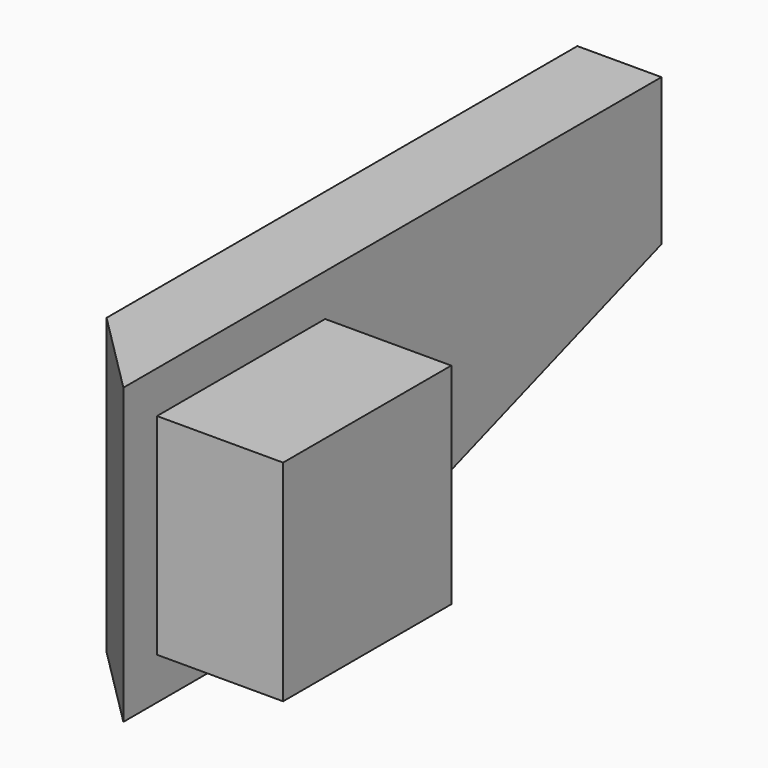
from build123d import *

# Parameters (mm, degrees)
F0_W     = 5
F0_H     = 5
F1_DEPTH = 3
F2_W     = 5
F2_H     = 5
F3_DEPTH = 2
F4_SIZE  = 1.99999


# Not quite as in the source:
# - a fillet or chamfer is up to 0.001 mm smaller than in the source, because OpenCascade refuses the exact size


with BuildPart() as f1:
    # F0 (on Right) → F1 (new body)
    with BuildSketch(Plane.YZ):
        with Locations((40.6040474772, 32.0952650385)):
            Rectangle(F0_W, F0_H)
    extrude(amount=F1_DEPTH)

    # F2 (on face) → F3 (join)
    with BuildSketch(Plane(origin=(0, 0, 0), x_dir=(0, -1, 0), z_dir=(-1, 0, 0))):
        with Locations((-40.6040474772, 32.0952650385)):
            Rectangle(F2_W, F2_H)
        Polygon((-37.1040474772, 28.5952650385), (-37.1040474772, 35.5952650385), (-43.1040474772, 35.5952650385), (-43.1040474772, 34.5952650385), (-38.1040474772, 34.5952650385), (-38.1040474772, 29.5952650385), (-43.1040474772, 29.5952650385), (-43.1040474772, 28.5952650385), align=None)
        Polygon((-43.1040474772, 34.5952650385), (-43.1040474772, 35.5952650385), (-51.1040474772, 32.7952650385), (-51.1040474772, 31.3952650385), (-43.1040474772, 28.5952650385), (-43.1040474772, 29.5952650385), align=None)
        Polygon((-51.1040474772, 32.7952650385), (-43.1040474772, 35.5952650385), (-51.1040474772, 35.5952650385), align=None)
        Polygon((-51.1040474772, 32.7952650385), (-51.1040474772, 35.5952650385), (-53.1040474772, 35.5952650385), (-53.1040474772, 32.0952650385), align=None)
        Polygon((-51.1040474772, 31.3952650385), (-51.1040474772, 32.7952650385), (-53.1040474772, 32.0952650385), align=None)
    extrude(amount=F3_DEPTH)

    # F4 (size 2 in the source; OpenCascade refuses exactly that, so slightly less here)
    f4_edges = [f1.edges().sort_by_distance(p)[0] for p in [
        (-2, 37.104047, 32.095265),
    ]]
    chamfer(f4_edges, length=F4_SIZE)


solid = f1.part
